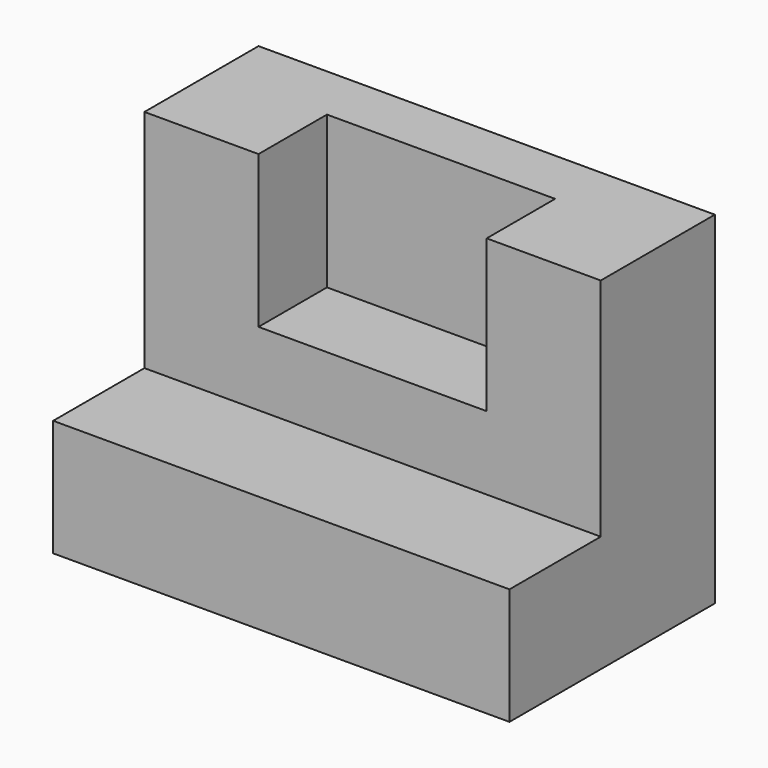
from build123d import *

# Parameters (mm, degrees)
F0_W     = 203.2
F0_H     = 152.4
F1_DEPTH = 25.4
F3_DEPTH = 38.1
F4_W     = 203.2
F4_H     = 51.9680035462
F5_DEPTH = 50.8


# Not quite as in the source:
# - a feature names something its author has since deleted; it is built from what else it names


with BuildPart() as f1:
    # F0 (on Front) → F1 (new body)
    with BuildSketch(Plane.XZ):
        with Locations((21.5330033839, 24.2319964538)):
            Rectangle(F0_W, F0_H)
    extrude(amount=F1_DEPTH)

    # F2 (on face) → F3 (join)
    with BuildSketch(Plane.XZ.offset(25.4)):
        Polygon((-29.2669966161, 32.6819717884), (-29.2669966161, 100.4319964538), (-80.0669966161, 100.4319964538), (-80.0669966161, -51.9680035462), (123.1330033839, -51.9680035462), (123.1330033839, 100.4319964538), (72.3330033839, 100.4319964538), (72.3330033839, 32.6819717884), align=None)
    extrude(amount=F3_DEPTH)

    # F4 (on face) → F5 (join)
    with BuildSketch(Plane.XZ.offset(63.5)):
        with Locations((21.5330033839, -25.9840017731)):
            Rectangle(F4_W, F4_H)
    extrude(amount=F5_DEPTH)


solid = f1.part
